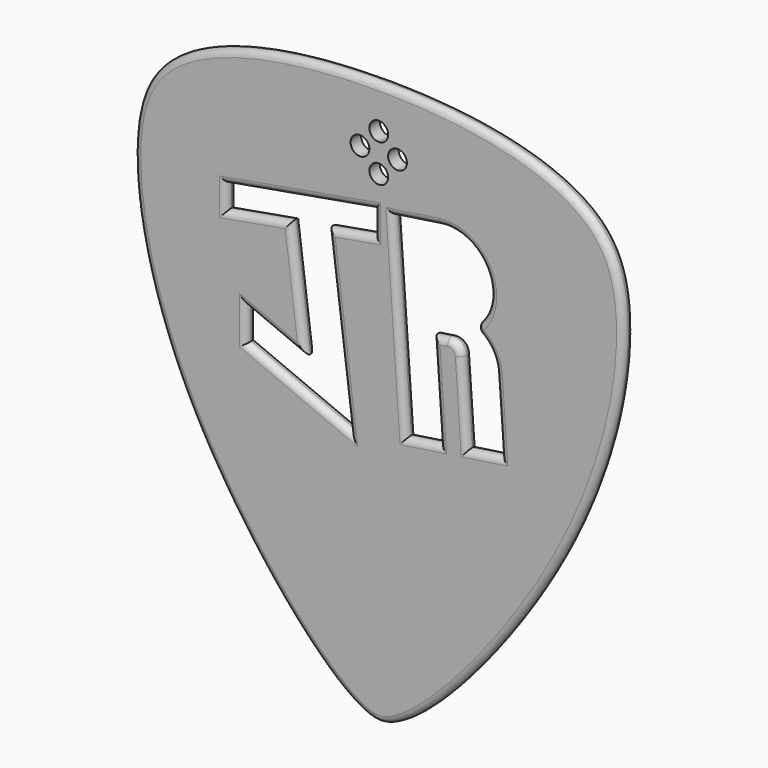
from build123d import *

# Parameters (mm, degrees)
F0_R     = 0.5
F1_DEPTH = 0.7
F2_R     = 0.3499
F3_R     = 0.34999


# Not quite as in the source:
# - a fillet or chamfer is up to 0.001 mm smaller than in the source, because OpenCascade refuses the exact size
# - a feature names something its author has since deleted; it is built from what else it names


with BuildPart() as f1:
    # F0 (on Front) → F1 (new body)
    with BuildSketch(Plane.XZ):
        with BuildLine():
            add(Edge.make_bspline(
                [(0, -23.25), (-2, -23.25), (-11.2052838081, -12.6454945316), (-13.7939030188, -0.3656097413), (-11.4819416014, 5.2828342286), (-5, 6.75), (0, 6.75)],
                knots=[0, 0, 0, 0, 0.2911366771, 0.5724636983, 0.7401439848, 1, 1, 1, 1], degree=3))
            add(Edge.make_bspline(
                [(0, -23.25), (2, -23.25), (11.2052838081, -12.6454945316), (13.7939030188, -0.3656097413), (11.4819416014, 5.2828342286), (5, 6.75), (0, 6.75)],
                knots=[0, 0, 0, 0, 0.2911366771, 0.5724636983, 0.7401439848, 1, 1, 1, 1], degree=3))
        make_face()
        Polygon((-0.25, -0.5), (-2.7097485316, -0.9337200319), (-1.542408067, -10.1097658164), (-7.0756138971, -7.7895000466), (-7.0756138971, -6.0395000466), (-3.9073137099, -7.3680785775), (-4.6816348886, -1.2814167995), (-8.1284620241, -1.8891854213), (-8.1284620241, -0.6391854213), (-0.25, 0.75), align=None, mode=Mode.SUBTRACT)
        with Locations((-1, 3.5)):
            Circle(F0_R, mode=Mode.SUBTRACT)
        with BuildLine():
            Line((1.4615160322, -9.4251533127), (0.75, 0.75))
            Line((0.75, 0.75), (3.2225739629, 1.1192939179))
            ThreePointArc((3.2225739629, 1.1192939179), (5.7434258747, -0.2851893969), (5.0276366561, -3.0807060821))
            ThreePointArc((5.0276366561, -3.0807060821), (5.868954756, -3.7604366774), (6.2333425349, -4.7788036907))
            Line((6.2333425349, -4.7788036907), (6.5055669166, -8.6717937201))
            Line((6.5055669166, -8.6717937201), (4.7253136633, -8.937685341))
            Line((4.7253136633, -8.937685341), (4.429349864, -4.7052058231))
            ThreePointArc((4.429349864, -4.7052058231), (4.1692268068, -4.2081365611), (3.6276527318, -4.0617146451))
            Line((3.6276527318, -4.0617146451), (2.8929869168, -4.1714414405))
            Line((2.8929869168, -4.1714414405), (3.2417692855, -9.1592616918))
            Line((3.2417692855, -9.1592616918), (1.4615160322, -9.4251533127))
        make_face(mode=Mode.SUBTRACT)
        with BuildLine():
            ThreePointArc((0.5, 2.5), (-0.3535533906, 2.1464466094), (0, 3))
            ThreePointArc((0, 3), (0.3535533906, 2.8535533906), (0.5, 2.5))
        make_face(mode=Mode.SUBTRACT)
        with BuildLine():
            ThreePointArc((1.5, 3.5), (1, 3), (0.5, 3.5))
            ThreePointArc((0.5, 3.5), (1, 4), (1.5, 3.5))
        make_face(mode=Mode.SUBTRACT)
        with BuildLine():
            ThreePointArc((0, 4), (-0.3535533906, 4.8535533906), (0.5, 4.5))
            ThreePointArc((0.5, 4.5), (0.3535533906, 4.1464466094), (0, 4))
        make_face(mode=Mode.SUBTRACT)
    extrude(amount=F1_DEPTH)

    # F2 (radius 0.35 in the source; OpenCascade refuses exactly that, so slightly less here)
    f2_edges = [f1.edges().sort_by_distance(p)[0] for p in [
        (-12.350697, -0.7, -5.69865),
        (12.350697, -0.7, -5.69865),
        (-12.350697, 0, -5.69865),
        (12.350697, 0, -5.69865),
    ]]
    fillet(f2_edges, radius=F2_R)

    # F3 (radius 0.35 in the source; OpenCascade refuses exactly that, so slightly less here)
    f3_edges = [f1.edges().sort_by_distance(p)[0] for p in [
        (-5.491464, -0.7, -6.703789),
        (-4.294474, -0.7, -4.324748),
        (-7.075614, -0.7, -6.9145),
        (-4.309011, -0.7, -8.949633),
        (-2.126078, -0.7, -5.521743),
        (-1.479874, -0.7, -0.71686),
        (-0.25, -0.7, 0.125),
        (-4.189231, -0.7, 0.055407),
        (-8.128462, -0.7, -1.264185),
        (-6.405048, -0.7, -1.585301),
        (1.986287, -0.7, 0.934647),
        (5.743426, -0.7, -0.285189),
        (1.105758, -0.7, -4.337577),
        (2.351643, -0.7, -9.292208),
        (3.067378, -0.7, -6.665352),
        (3.26032, -0.7, -4.116578),
        (5.61544, -0.7, -8.80474),
        (6.369455, -0.7, -6.725299),
        (5.868955, -0.7, -3.760437),
        (5.61544, 0, -8.80474),
        (4.577332, 0, -6.821446),
        (6.369455, 0, -6.725299),
        (5.743426, 0, -0.285189),
        (1.986287, 0, 0.934647),
        (1.105758, 0, -4.337577),
        (3.26032, 0, -4.116578),
        (3.067378, 0, -6.665352),
        (2.351643, 0, -9.292208),
        (-2.126078, 0, -5.521743),
        (-4.309011, 0, -8.949633),
        (-7.075614, 0, -6.9145),
        (-5.491464, 0, -6.703789),
        (-4.294474, 0, -4.324748),
        (-6.405048, 0, -1.585301),
        (-8.128462, 0, -1.264185),
        (-4.189231, 0, 0.055407),
        (-1.479874, 0, -0.71686),
        (-0.25, 0, 0.125),
        (5.027637, -0.35, -3.080706),
    ]]
    fillet(f3_edges, radius=F3_R)


solid = f1.part
